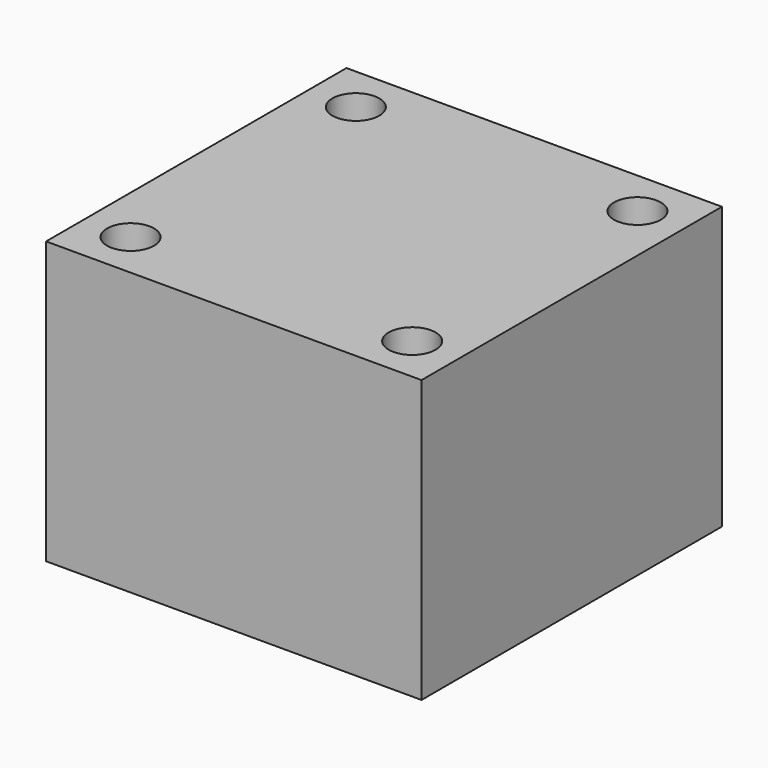
from build123d import *

# Parameters (mm, degrees)
F0_W     = 50.8
F0_H     = 50.8
F0_R     = 3.175
F1_DEPTH = 19.05


# Not quite as in the source:
# - the program builds the solid bodies; features that only make, move or delete a surface that nothing else refers to are left out


with BuildPart() as f1:
    # F0 (on Top) → F1 (new body, symmetric)
    with BuildSketch(Plane.XY):
        Rectangle(F0_W, F0_H)
        with Locations((-19.05, -19.05)):
            Circle(F0_R, mode=Mode.SUBTRACT)
        with Locations((19.05, -19.05)):
            Circle(F0_R, mode=Mode.SUBTRACT)
        with Locations((-19.05, 19.05)):
            Circle(F0_R, mode=Mode.SUBTRACT)
        with Locations((19.05, 19.05)):
            Circle(F0_R, mode=Mode.SUBTRACT)
    extrude(amount=F1_DEPTH, both=True)


solid = f1.part
